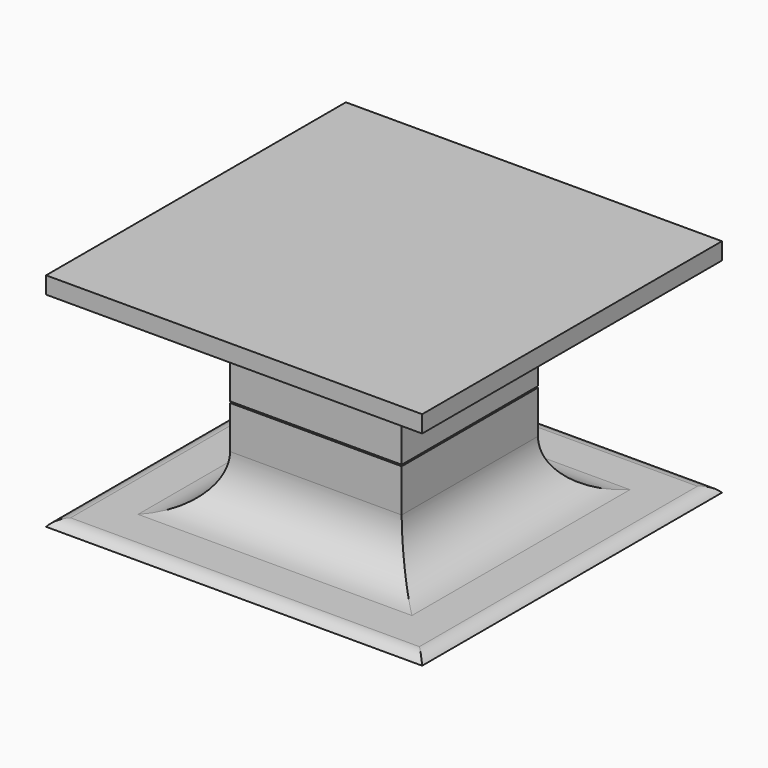
from build123d import *

# Parameters (mm, degrees)
F0_W         = 110.4
F0_H         = 110
F0_W_2       = 50.4
F0_H_2       = 50
F0_W_3       = 44.4
F0_H_3       = 44
F1_DEPTH     = 2
F2_DEPTH     = 30
F3_DEPTH     = 30
F4_DEPTH     = 0.5
F5_START     = 60
F5_DEPTH     = 5
F6_R         = 15
F6_2_R       = 15
F7_T1_DEPTH  = 130.4
F7_T3_DEPTH  = 130
F8_T1_DEPTH  = 44
F8_T3_DEPTH  = 44.4
F8_T9_DEPTH  = 56.9
F8_T15_DEPTH = 56.5
F8_T24_DEPTH = 56.9
F8_T30_DEPTH = 56.5
F8_T39_DEPTH = 56.5
F8_T45_DEPTH = 56.9
F8_T54_DEPTH = 56.9
F8_T60_DEPTH = 56.5


# Not quite as in the source:
# - a fillet or chamfer that OpenCascade refuses, or shapes differently, is made with other operations: its cross-section is extruded or revolved along the edge and cut away or added


with BuildPart() as f1:
    # F0 (on Top) → F1 (new body)
    with BuildSketch(Plane.XY):
        Rectangle(F0_W, F0_H)
        Rectangle(F0_W_2, F0_H_2, mode=Mode.SUBTRACT)
        Rectangle(F0_W_2, F0_H_2)
        Rectangle(F0_W_3, F0_H_3, mode=Mode.SUBTRACT)
    extrude(amount=F1_DEPTH)

    # F0 (on Top) → F2 (join)
    with BuildSketch(Plane.XY):
        Rectangle(F0_W_2, F0_H_2)
        Rectangle(F0_W_3, F0_H_3, mode=Mode.SUBTRACT)
    extrude(amount=F2_DEPTH)


with BuildPart() as f3:
    # F3 (new): a face of the model
    f3_faces = [f1.part.faces().sort_by_distance(p)[0] for p in [
        (24.4900591574, 0, 30),
    ]]
    extrude(f3_faces, amount=F3_DEPTH)

    # F0 (on Top) → F5 (join)
    with BuildSketch(Plane.XY.offset(F5_START)):
        Rectangle(F0_W, F0_H)
        Rectangle(F0_W_2, F0_H_2, mode=Mode.SUBTRACT)
        Rectangle(F0_W_2, F0_H_2)
        Rectangle(F0_W_3, F0_H_3, mode=Mode.SUBTRACT)
        Rectangle(F0_W_3, F0_H_3)
    extrude(amount=F5_DEPTH)

    # F6#2
    f6_2_edges = [f3.edges().sort_by_distance(p)[0] for p in [
        (0, -25, 60),
        (-25.2, 0, 60),
        (0, 25, 60),
        (25.2, 0, 60),
    ]]
    fillet(f6_2_edges, radius=F6_2_R)


with BuildPart() as f1_1:
    add(f1.part)

    # F0 (on Top) → F4 (join)
    with BuildSketch(Plane.XY):
        Rectangle(F0_W_3, F0_H_3)
    extrude(amount=F4_DEPTH)

    # F6
    f6_edges = [f1_1.edges().sort_by_distance(p)[0] for p in [
        (25.2, 0, 2),
        (0, -25, 2),
        (-25.2, 0, 2),
        (0, 25, 2),
    ]]
    fillet(f6_edges, radius=F6_R)

    # F7: fillet of radius 5 on 4 edges, made by hand

    # F7_s2 → F7_t1 (cut)
    with BuildSketch(Plane.YZ.offset(-65.2)):
        with BuildLine():
            ThreePointArc((51, 2), (53.2360679775, 1.472135955), (55, 0))
            Line((55, 0), (55, 2))
            Line((55, 2), (51, 2))
        make_face()
        with BuildLine():
            ThreePointArc((-51, 2), (-53.2360679775, 1.472135955), (-55, 0))
            Line((-55, 0), (-55, 2))
            Line((-55, 2), (-51, 2))
        make_face()
    extrude(amount=F7_T1_DEPTH, mode=Mode.SUBTRACT)

    # F7_s4 → F7_t3 (cut)
    with BuildSketch(Plane.XZ.offset(-65)):
        with BuildLine():
            ThreePointArc((51.2, 2), (53.4360679775, 1.472135955), (55.2, 0))
            Line((55.2, 0), (55.2, 2))
            Line((55.2, 2), (51.2, 2))
        make_face()
        with BuildLine():
            ThreePointArc((-51.2, 2), (-53.4360679775, 1.472135955), (-55.2, 0))
            Line((-55.2, 0), (-55.2, 2))
            Line((-55.2, 2), (-51.2, 2))
        make_face()
    extrude(amount=F7_T3_DEPTH, mode=Mode.SUBTRACT)

    # F8: fillet of radius 5 on 4 edges, made by hand

    # F8_s2 → F8_t1 (cut)
    with BuildSketch(Plane.XZ.offset(-22)):
        with BuildLine():
            ThreePointArc((-27.2, 30), (-23.6644660941, 28.5355339059), (-22.2, 25))
            Line((-22.2, 25), (-22.2, 30))
            Line((-22.2, 30), (-27.2, 30))
        make_face()
        with BuildLine():
            ThreePointArc((27.2, 30), (23.6644660941, 28.5355339059), (22.2, 25))
            Line((22.2, 25), (22.2, 30))
            Line((22.2, 30), (27.2, 30))
        make_face()
    extrude(amount=F8_T1_DEPTH, mode=Mode.SUBTRACT)

    # F8_s4 → F8_t3 (cut)
    with BuildSketch(Plane.YZ.offset(-22.2)):
        with BuildLine():
            ThreePointArc((-27, 30), (-23.4644660941, 28.5355339059), (-22, 25))
            Line((-22, 25), (-22, 30))
            Line((-22, 30), (-27, 30))
        make_face()
        with BuildLine():
            ThreePointArc((27, 30), (23.4644660941, 28.5355339059), (22, 25))
            Line((22, 25), (22, 30))
            Line((22, 30), (27, 30))
        make_face()
    extrude(amount=F8_T3_DEPTH, mode=Mode.SUBTRACT)


with BuildPart() as f8_tool7:
    # F8_s8 → F8_t9 (new body)
    with BuildSketch(Plane.YZ.offset(22.2)):
        with BuildLine():
            ThreePointArc((-27, 30), (-23.4644660941, 28.5355339059), (-22, 25))
            Line((-22, 25), (-22, 30))
            Line((-22, 30), (-27, 30))
        make_face()
    extrude(amount=-F8_T9_DEPTH)

    split(bisect_by=Plane.XZ.offset(25), keep=Keep.BOTTOM)

    split(bisect_by=Plane.YZ.offset(-25.2), keep=Keep.TOP)

    split(bisect_by=Plane.YZ.offset(-22.2), keep=Keep.BOTTOM)


with BuildPart() as f8_tool13:
    # F8_s14 → F8_t15 (new body)
    with BuildSketch(Plane.XZ.offset(34.5)):
        with BuildLine():
            ThreePointArc((-27.2, 30), (-23.6644660941, 28.5355339059), (-22.2, 25))
            Line((-22.2, 25), (-22.2, 30))
            Line((-22.2, 30), (-27.2, 30))
        make_face()
    extrude(amount=-F8_T15_DEPTH)

    split(bisect_by=Plane.XZ.offset(25), keep=Keep.BOTTOM)

    split(bisect_by=Plane.YZ.offset(-25.2), keep=Keep.TOP)

    split(bisect_by=Plane.XZ.offset(22), keep=Keep.TOP)


with BuildPart() as f8_tool7_1:
    add(f8_tool7.part)

    # F8_t19: intersect F8_tool13
    add(f8_tool13.part, mode=Mode.INTERSECT)


with BuildPart() as f1_2:
    add(f1_1.part)

    # F8_t5: cut F8_tool7
    add(f8_tool7_1.part, mode=Mode.SUBTRACT)


with BuildPart() as f8_tool22:
    # F8_s23 → F8_t24 (new body)
    with BuildSketch(Plane.YZ.offset(-34.7)):
        with BuildLine():
            ThreePointArc((27, 30), (23.4644660941, 28.5355339059), (22, 25))
            Line((22, 25), (22, 30))
            Line((22, 30), (27, 30))
        make_face()
    extrude(amount=F8_T24_DEPTH)

    split(bisect_by=Plane.XZ.offset(-25), keep=Keep.TOP)

    split(bisect_by=Plane.YZ.offset(-25.2), keep=Keep.TOP)

    split(bisect_by=Plane.YZ.offset(-22.2), keep=Keep.BOTTOM)


with BuildPart() as f8_tool28:
    # F8_s29 → F8_t30 (new body)
    with BuildSketch(Plane.XZ.offset(22)):
        with BuildLine():
            ThreePointArc((-27.2, 30), (-23.6644660941, 28.5355339059), (-22.2, 25))
            Line((-22.2, 25), (-22.2, 30))
            Line((-22.2, 30), (-27.2, 30))
        make_face()
    extrude(amount=-F8_T30_DEPTH)

    split(bisect_by=Plane.XZ.offset(-25), keep=Keep.TOP)

    split(bisect_by=Plane.YZ.offset(-25.2), keep=Keep.TOP)

    split(bisect_by=Plane.XZ.offset(-22), keep=Keep.BOTTOM)


with BuildPart() as f8_tool22_1:
    add(f8_tool22.part)

    # F8_t34: intersect F8_tool28
    add(f8_tool28.part, mode=Mode.INTERSECT)


with BuildPart() as f1_3:
    add(f1_2.part)

    # F8_t20: cut F8_tool22
    add(f8_tool22_1.part, mode=Mode.SUBTRACT)


with BuildPart() as f8_tool37:
    # F8_s38 → F8_t39 (new body)
    with BuildSketch(Plane.XZ.offset(-22)):
        with BuildLine():
            ThreePointArc((27.2, 30), (23.6644660941, 28.5355339059), (22.2, 25))
            Line((22.2, 25), (22.2, 30))
            Line((22.2, 30), (27.2, 30))
        make_face()
    extrude(amount=F8_T39_DEPTH)

    split(bisect_by=Plane.YZ.offset(25.2), keep=Keep.BOTTOM)

    split(bisect_by=Plane.XZ.offset(25), keep=Keep.BOTTOM)

    split(bisect_by=Plane.XZ.offset(22), keep=Keep.TOP)


with BuildPart() as f8_tool43:
    # F8_s44 → F8_t45 (new body)
    with BuildSketch(Plane.YZ.offset(34.7)):
        with BuildLine():
            ThreePointArc((-27, 30), (-23.4644660941, 28.5355339059), (-22, 25))
            Line((-22, 25), (-22, 30))
            Line((-22, 30), (-27, 30))
        make_face()
    extrude(amount=-F8_T45_DEPTH)

    split(bisect_by=Plane.YZ.offset(25.2), keep=Keep.BOTTOM)

    split(bisect_by=Plane.XZ.offset(25), keep=Keep.BOTTOM)

    split(bisect_by=Plane.YZ.offset(22.2), keep=Keep.TOP)


with BuildPart() as f8_tool37_1:
    add(f8_tool37.part)

    # F8_t49: intersect F8_tool43
    add(f8_tool43.part, mode=Mode.INTERSECT)


with BuildPart() as f1_4:
    add(f1_3.part)

    # F8_t35: cut F8_tool37
    add(f8_tool37_1.part, mode=Mode.SUBTRACT)


with BuildPart() as f8_tool52:
    # F8_s53 → F8_t54 (new body)
    with BuildSketch(Plane.YZ.offset(-22.2)):
        with BuildLine():
            ThreePointArc((27, 30), (23.4644660941, 28.5355339059), (22, 25))
            Line((22, 25), (22, 30))
            Line((22, 30), (27, 30))
        make_face()
    extrude(amount=F8_T54_DEPTH)

    split(bisect_by=Plane.YZ.offset(25.2), keep=Keep.BOTTOM)

    split(bisect_by=Plane.XZ.offset(-25), keep=Keep.TOP)

    split(bisect_by=Plane.YZ.offset(22.2), keep=Keep.TOP)


with BuildPart() as f8_tool58:
    # F8_s59 → F8_t60 (new body)
    with BuildSketch(Plane.XZ.offset(-34.5)):
        with BuildLine():
            ThreePointArc((27.2, 30), (23.6644660941, 28.5355339059), (22.2, 25))
            Line((22.2, 25), (22.2, 30))
            Line((22.2, 30), (27.2, 30))
        make_face()
    extrude(amount=F8_T60_DEPTH)

    split(bisect_by=Plane.YZ.offset(25.2), keep=Keep.BOTTOM)

    split(bisect_by=Plane.XZ.offset(-25), keep=Keep.TOP)

    split(bisect_by=Plane.XZ.offset(-22), keep=Keep.BOTTOM)


with BuildPart() as f8_tool52_1:
    add(f8_tool52.part)

    # F8_t64: intersect F8_tool58
    add(f8_tool58.part, mode=Mode.INTERSECT)


with BuildPart() as f1_5:
    add(f1_4.part)

    # F8_t50: cut F8_tool52
    add(f8_tool52_1.part, mode=Mode.SUBTRACT)


solid = Compound([f3.part, f1_5.part])
